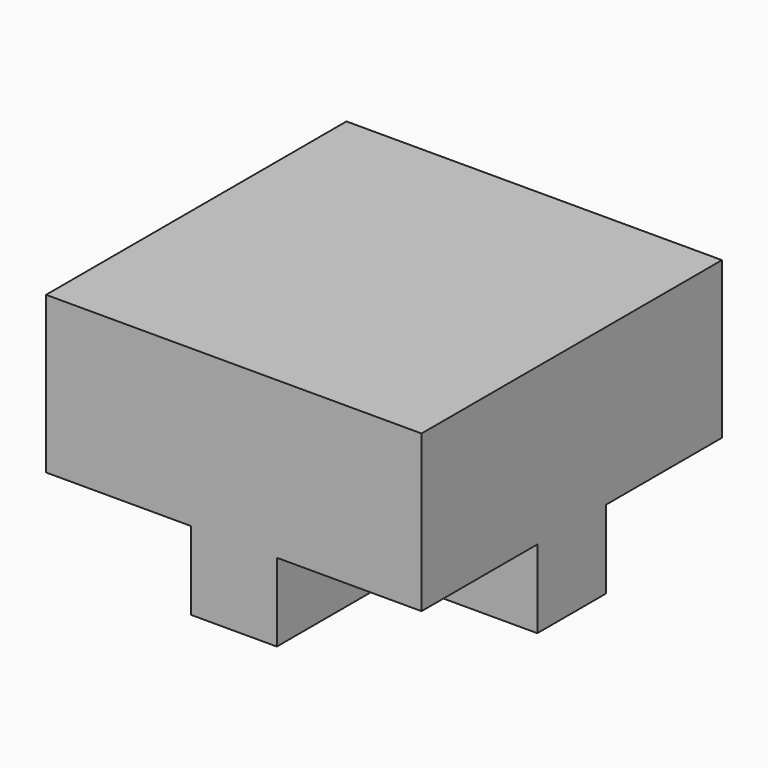
from build123d import *

# Parameters (mm, degrees)
F0_W     = 5.5
F0_H     = 8
F1_DEPTH = 5
F0_R     = 1
F2_COUNT = 4
F4_W     = 5.5
F4_H     = 8
F4_W_2   = 8
F4_H_2   = 5.5
F5_DEPTH = 10


with BuildPart() as f1:
    # F0 (on Top) → F1 (new body)
    with BuildSketch(Plane.XY):
        with Locations((0, 8)):
            Rectangle(F0_W, F0_H)
    extrude(amount=F1_DEPTH)


with BuildPart() as f1b:
    # F0 (on Top) → F1, piece 2 (new body)
    with BuildSketch(Plane.XY):
        Circle(F0_R)
    extrude(amount=F1_DEPTH)


with BuildPart() as f2_1:
    # F2: instance of F1
    add(f1.part.rotate(Axis((0, 0, 0), (0, 0, -1)), 1 * 360 / F2_COUNT))


with BuildPart() as f2_2:
    # F2: instance of F1
    add(f1.part.rotate(Axis((0, 0, 0), (0, 0, -1)), 2 * 360 / F2_COUNT))


with BuildPart() as f2_3:
    # F2: instance of F1
    add(f1.part.rotate(Axis((0, 0, 0), (0, 0, -1)), 3 * 360 / F2_COUNT))


with BuildPart() as f1_1:
    add(f1.part)

    add(f2_1.part)  # F5 merges F2_1

    add(f2_2.part)  # F5 merges F2_2

    add(f2_3.part)  # F5 merges F2_3
    # F4 (on face) → F5 (join)
    with BuildSketch(Plane.XY.offset(5)):
        with Locations((0, 8)):
            Rectangle(F4_W, F4_H)
        Polygon((12, 12), (2.75, 12), (2.75, 4), (-2.75, 4), (-2.75, 12), (-12, 12), (-12, 2.75), (-4, 2.75), (-4, -2.75), (-12, -2.75), (-12, -12), (-2.75, -12), (-2.75, -4), (2.75, -4), (2.75, -12), (12, -12), (12, -2.75), (4, -2.75), (4, 2.75), (12, 2.75), align=None)
        with Locations((8, 0)):
            Rectangle(F4_W_2, F4_H_2)
        with Locations((-8, 0)):
            Rectangle(F4_W_2, F4_H_2)
        with Locations((0, -8)):
            Rectangle(F4_W, F4_H)
    extrude(amount=F5_DEPTH)


solid = f1_1.part
